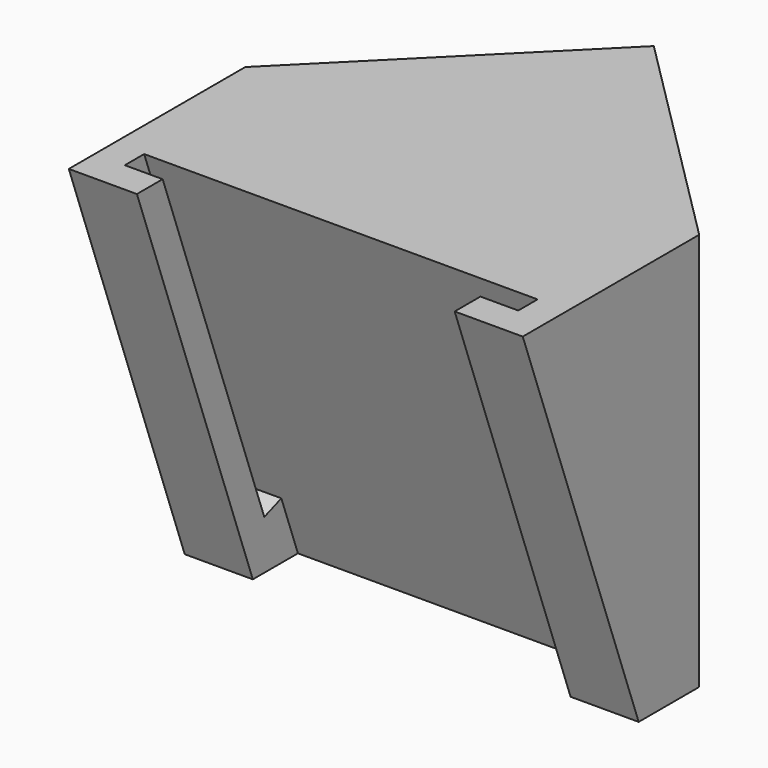
from build123d import *

# Parameters (mm, degrees)
F1_DEPTH = 15
F2_DEPTH = 13
F3_DEPTH = 10.5
F4_DEPTH = 10.5
F6_DEPTH = 30


with BuildPart() as f1:
    # F0 (on Right) → F1 (new body, symmetric)
    with BuildSketch(Plane.YZ):
        Polygon((-24.5765640131, 26.311393382), (-15, 0), (-12.871644455, 0), (-14.0529973008, 3.2457402682), (-22.4482084682, 26.311393382), align=None)
        Polygon((-22.4482084682, 26.311393382), (-14.0529973008, 3.2457402682), (-12.6434583696, 3.7587704831), (-20.8519418095, 26.311393382), align=None)
        Polygon((-14.0529973008, 3.2457402682), (-12.871644455, 0), (-11.2753777963, 0), (-12.6434583696, 3.7587704831), align=None)
        Polygon((-12.6434583696, 3.7587704831), (-11.2753777963, 0), (15, 0), (15, 26.311393382), (-20.8519418095, 26.311393382), align=None)
    extrude(amount=F1_DEPTH, both=True)

    # F0 (on Right) → F2 (cut, symmetric)
    with BuildSketch(Plane.YZ):
        Polygon((-22.4482084682, 26.311393382), (-14.0529973008, 3.2457402682), (-12.6434583696, 3.7587704831), (-20.8519418095, 26.311393382), align=None)
    extrude(amount=F2_DEPTH, both=True, mode=Mode.SUBTRACT)

    # F0 (on Right) → F3 (cut, symmetric)
    with BuildSketch(Plane.YZ):
        Polygon((-24.5765640131, 26.311393382), (-15, 0), (-12.871644455, 0), (-14.0529973008, 3.2457402682), (-22.4482084682, 26.311393382), align=None)
    extrude(amount=F3_DEPTH, both=True, mode=Mode.SUBTRACT)

    # F0 (on Right) → F4 (cut, symmetric)
    with BuildSketch(Plane.YZ):
        Polygon((-14.0529973008, 3.2457402682), (-12.871644455, 0), (-11.2753777963, 0), (-12.6434583696, 3.7587704831), align=None)
    extrude(amount=F4_DEPTH, both=True, mode=Mode.SUBTRACT)

    # F5 (on face) → F6 (cut)
    with BuildSketch(Plane(origin=(0, 0, 0), x_dir=(1, 0, 0), z_dir=(0, 0, -1))):
        Polygon((0, -5), (-15, 10), (-15, -15), (15, -15), (15, 10), align=None)
    extrude(amount=-F6_DEPTH, mode=Mode.SUBTRACT)


solid = f1.part
